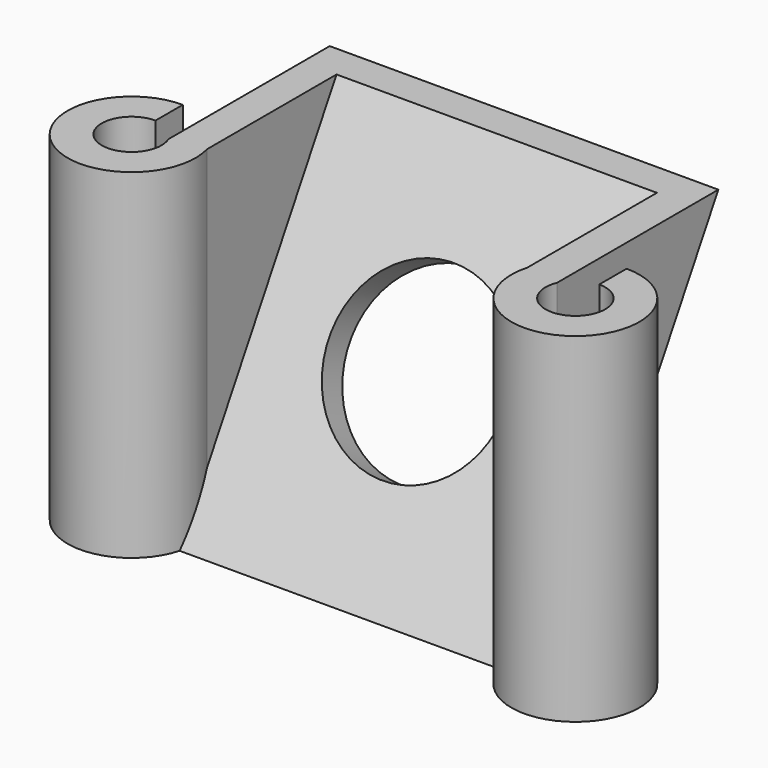
from build123d import *

# Parameters (mm, degrees)
F0_R      = 3.75
F0_R_2    = 1.75
F1_DEPTH  = 19.9
F2_W      = 18.7715838526
F2_H      = 2
F5_W      = 18.7715838526
F5_H      = 2
F8_R      = 5.25
F9_DEPTH  = 11.6830509442
F11_DEPTH = 2
F12_W     = 1.6142080737
F12_H     = 6.9905174896
F13_DEPTH = 19.9010001


# Not quite as in the source:
# - a pattern or mirror of a feature is missing from the dataset's text; its kind, count and spacing are read off the source's solid


with BuildPart() as f1:
    # F0 (on Top) → F1 (new body)
    with BuildSketch(Plane.XY):
        with Locations((13, 0)):
            Circle(F0_R)
        with Locations((13, 0)):
            Circle(F0_R_2, mode=Mode.SUBTRACT)
    extrude(amount=F1_DEPTH)



with BuildPart() as f1b:
    # F0 (on Top) → F1, piece 2 (new body)
    with BuildSketch(Plane.XY):
        with Locations((-13, 0)):
            Circle(F0_R)
        with Locations((-13, 0)):
            Circle(F0_R_2, mode=Mode.SUBTRACT)
    extrude(amount=F1_DEPTH)


with BuildPart() as f1_1:
    add(f1.part)

    add(f1b.part)  # F6 merges F1b
    # F2 (on Top) → F6 section 0
    with BuildSketch(Plane.XY):
        Rectangle(F2_W, F2_H)
    # F5 (on offset) → F6 section 1
    with BuildSketch(Plane.XY.offset(19.9)):
        with Locations((0, 11.4892703569)):
            Rectangle(F5_W, F5_H)
    loft()

    # F8 (on offset) → F9 (cut, through all)
    with BuildSketch(Plane(origin=(0, -0.75, 0.4330127019), x_dir=(1, 0, 0), z_dir=(0, -0.8660254038, 0.5))):
        with Locations((0, 10.9892703569)):
            Circle(F8_R)
    extrude(amount=-F9_DEPTH, mode=Mode.SUBTRACT)

    # F10 (on face) → F11 (join)
    with BuildSketch(Plane(origin=(-9.3857919263, 0, 0), x_dir=(0, -1, 0), z_dir=(-1, 0, 0))):
        Polygon((-1, 19.9), (-12.4892703569, 19.9), (-1, 0), (-1, 3.4641016151), align=None)
    f11 = extrude(amount=F11_DEPTH)

    # F11_copies: F11 across plane
    add(f11.mirror(Plane(origin=(0, 0, 0), x_dir=(0, 0, 1), z_dir=(1, 0, 0))))

    # F12 (on Top) → F13 (cut, through all)
    with BuildSketch(Plane.XY):
        with Locations((-12.1928959631, 3.4952587448)):
            Rectangle(F12_W, F12_H)
    f13 = extrude(amount=F13_DEPTH, mode=Mode.SUBTRACT)

    # F13_copies: F13 across plane
    add(f13.mirror(Plane(origin=(0, 0, 0), x_dir=(0, 0, 1), z_dir=(1, 0, 0))), mode=Mode.SUBTRACT)


solid = f1_1.part
